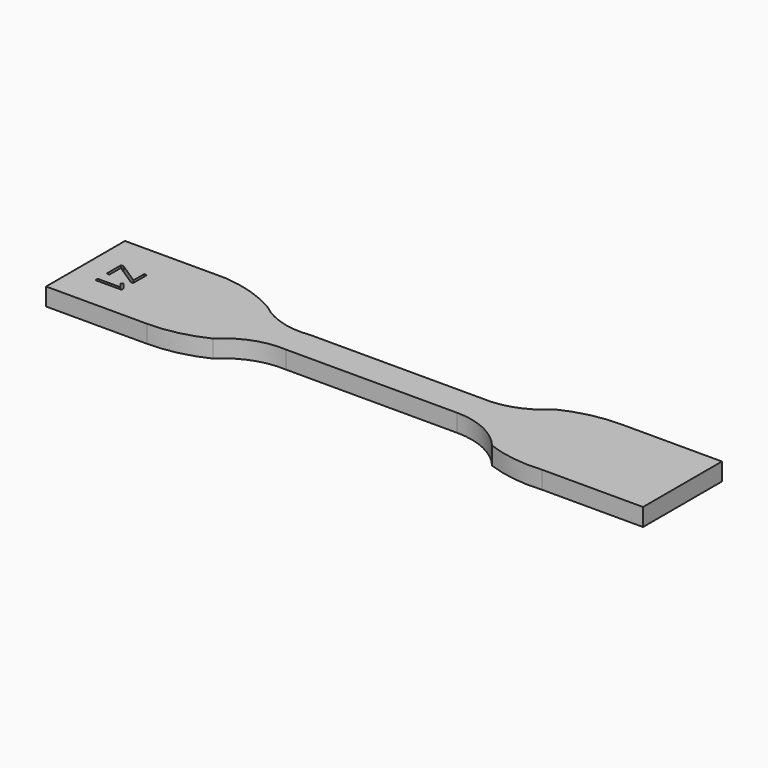
from build123d import *

# Parameters (mm, degrees)
F1_DEPTH     = 3.4
F2_TEXT_SIZE = 7.0564552314
F3_DEPTH     = 1


# Not quite as in the source:
# - Text() gives the source's letters only with a copy of the font that has no kerning and outlines rounded to 1/6400 em; it was checked with that copy


with BuildPart() as f1:
    # F0 (on Top) → F1 (new body)
    with BuildSketch(Plane.XY):
        with BuildLine():
            Line((-14.4320548165, 19.7811394548), (-33.8720548165, 19.7811394548))
            Line((-33.8720548165, 19.7811394548), (-33.8720548165, 0.7811394548))
            Line((-33.8720548165, 0.7811394548), (-14.4320548165, 0.7811394548))
            ThreePointArc((-14.4320548165, 0.7811394548), (-8.9053122052, 1.3996892086), (-3.6520548165, 3.2247301661))
            ThreePointArc((-3.6520548165, 3.2247301661), (1.3014698263, 6.4128780055), (7.1279451835, 7.2811394548))
            Line((7.1279451835, 7.2811394548), (40.1279451835, 7.2811394548))
            ThreePointArc((40.1279451835, 7.2811394548), (46.0837574042, 5.9511158081), (50.9079451835, 2.2137538538))
            ThreePointArc((50.9079451835, 2.2137538538), (56.2191047011, 0.9041953221), (61.6879451835, 0.7811394548))
            Line((61.6879451835, 0.7811394548), (81.1279451835, 0.7811394548))
            Line((81.1279451835, 0.7811394548), (81.1279451835, 19.7811394548))
            Line((81.1279451835, 19.7811394548), (61.6879451835, 19.7811394548))
            ThreePointArc((61.6879451835, 19.7811394548), (56.1612025723, 19.162589701), (50.9079451835, 17.3375487435))
            ThreePointArc((50.9079451835, 17.3375487435), (45.9544205407, 14.1494009041), (40.1279451835, 13.2811394548))
            Line((40.1279451835, 13.2811394548), (7.1279451835, 13.2811394548))
            ThreePointArc((7.1279451835, 13.2811394548), (1.4167452884, 13.6925537245), (-3.6520548165, 16.3560723447))
            ThreePointArc((-3.6520548165, 16.3560723447), (-8.8458057958, 18.686276846), (-14.4320548165, 19.7811394548))
        make_face()
    extrude(amount=F1_DEPTH)

    # F2 (on face) → F3 (cut)
    with BuildSketch(Plane.XY.offset(3.4)):
        with Locations(Location((-29.3886531144, 13.5272191837), (0, 0, -90))):
            Text('Z1', F2_TEXT_SIZE, font='Open Sans', text_align=(TextAlign.LEFT, TextAlign.BOTTOM))
    extrude(amount=-F3_DEPTH, mode=Mode.SUBTRACT)


solid = f1.part
